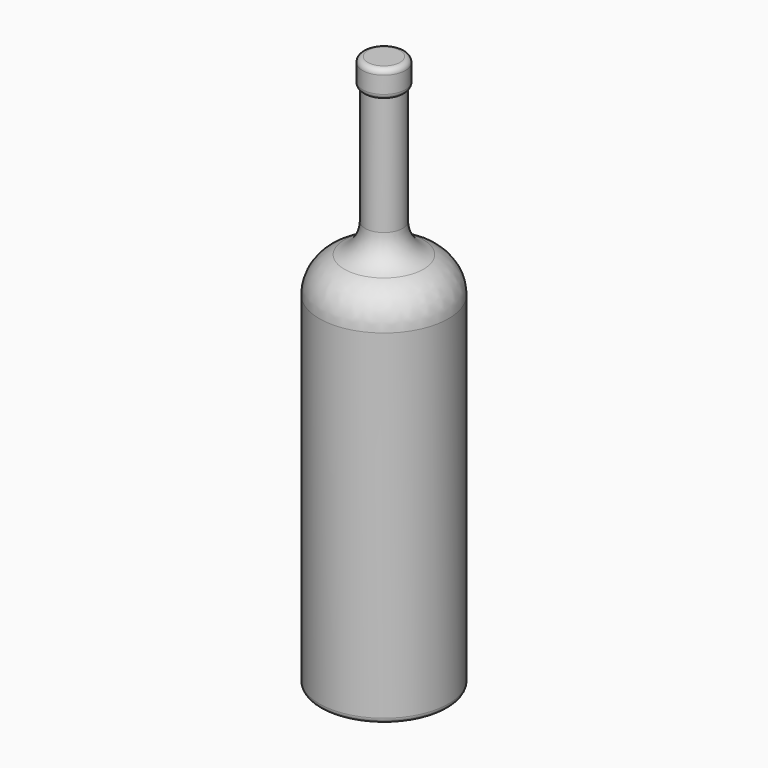
from build123d import *

# Parameters (mm, degrees)
F0_W   = 1.5875
F0_H   = 15.875
F0_W_2 = 11.1125
F0_H_2 = 69.85


# Not quite as in the source:
# - a fillet or chamfer that OpenCascade refuses, or shapes differently, is made with other operations: its cross-section is extruded or revolved along the edge and cut away or added


with BuildPart() as f1:
    # F0 (on Front) → F1 (revolve)
    with BuildSketch(Plane.XZ):
        with Locations((-11.90625, 217.4875)):
            Rectangle(F0_W, F0_H)
        with Locations((-5.55625, 217.4875)):
            Rectangle(F0_W_2, F0_H)
        with Locations((-5.55625, 174.625)):
            Rectangle(F0_W_2, F0_H_2)
        with BuildLine():
            Line((-38.1, 101.6), (0, 101.6))
            Line((0, 101.6), (0, 139.7))
            Line((0, 139.7), (-11.1125, 139.7))
            ThreePointArc((-11.1125, 139.7), (-14.586457312, 129.203622534), (-23.4018713236, 122.5304827094))
            ThreePointArc((-23.4018713236, 122.5304827094), (-34.0584362623, 114.387885801), (-38.1, 101.6))
        make_face()
        with BuildLine():
            Line((0, -85.043540958), (0, 101.6))
            Line((0, 101.6), (-38.1, 101.6))
            Line((-38.1, 101.6), (-38.1, -101.6))
            Line((-38.1, -101.6), (-24.4468970238, -101.6))
            ThreePointArc((-24.4468970238, -101.6), (-18.8855290947, -99.8940128678), (-15.2374166451, -95.3629554974))
            ThreePointArc((-15.2374166451, -95.3629554974), (-9.2014833377, -87.8661580499), (0, -85.043540958))
        make_face()
    revolve(axis=Axis((0, 0, 70.190729521), (0, 0, 1)))

    # F2: fillet of radius 3.175 on 3 edges, made by hand

    # F2_s1 → F2_t2 (revolve, cut)
    with BuildSketch(Plane.XZ):
        with BuildLine():
            ThreePointArc((-38.1, -98.425), (-37.1700640303, -100.6700640303), (-34.925, -101.6))
            Line((-34.925, -101.6), (-34.925, -101.6635))
            Line((-34.925, -101.6635), (-38.1635, -101.6635))
            Line((-38.1635, -101.6635), (-38.1635, -98.425))
            Line((-38.1635, -98.425), (-38.1, -98.425))
        make_face()
    revolve(axis=Axis((0, 0, -101.6), (0, 0, 1)), mode=Mode.SUBTRACT)

    # F2_s3 → F2_t4 (revolve, cut)
    with BuildSketch(Plane.XZ):
        with BuildLine():
            ThreePointArc((-9.525, 225.425), (-11.7700640303, 224.4950640303), (-12.7, 222.25))
            Line((-12.7, 222.25), (-12.7635, 222.25))
            Line((-12.7635, 222.25), (-12.7635, 225.4885))
            Line((-12.7635, 225.4885), (-9.525, 225.4885))
            Line((-9.525, 225.4885), (-9.525, 225.425))
        make_face()
    revolve(axis=Axis((0, 0, 225.425), (0, 0, 1)), mode=Mode.SUBTRACT)

    # F2_s5 → F2_t6 (revolve, cut)
    with BuildSketch(Plane.XZ):
        with BuildLine():
            ThreePointArc((-11.1125, 209.55), (-12.274630657, 210.712130657), (-12.7, 212.299630657))
            Line((-12.7, 212.299630657), (-12.7635, 212.299630657))
            Line((-12.7635, 212.299630657), (-12.7635, 209.55))
            Line((-12.7635, 209.55), (-12.7, 209.4865))
            ThreePointArc((-12.7, 209.4865), (-11.90625, 209.4865), (-11.14425, 209.4950073869))
            Line((-11.14425, 209.4950073869), (-11.1125, 209.55))
        make_face()
    revolve(axis=Axis((0, 0, 209.55), (0, 0, 1)), mode=Mode.SUBTRACT)


solid = f1.part
